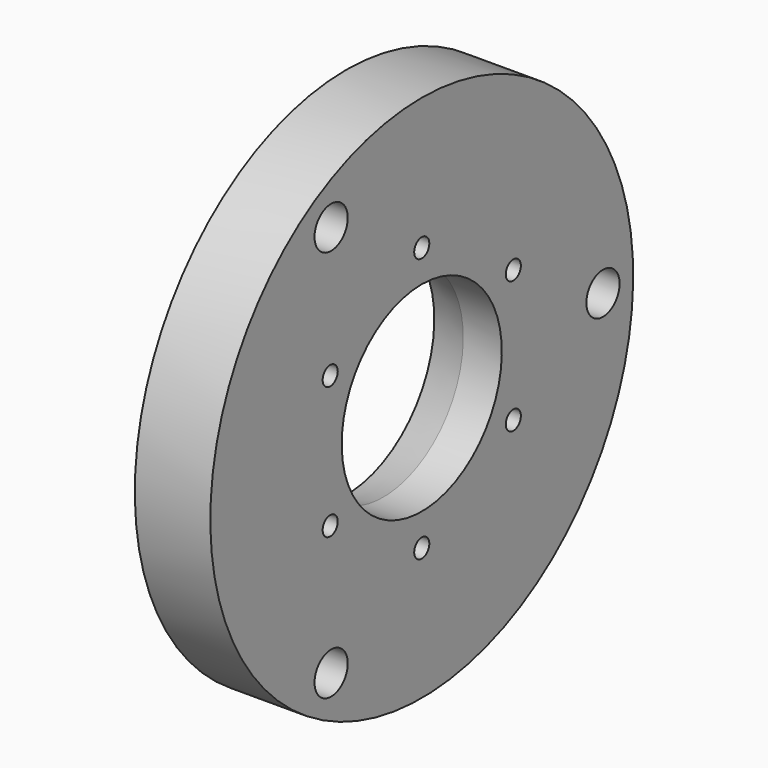
from build123d import *

# Parameters (mm, degrees)
F2_R            = 5.5
F3_DEPTH        = 20.001
F3_COPIES_COUNT = 3
F4_R            = 2.5
F5_DEPTH        = 15
F5_COPIES_COUNT = 6


# Not quite as in the source:
# - a pattern or mirror of a feature is missing from the dataset's text; its kind, count and spacing are read off the source's solid


with BuildPart() as f1:
    # F0 (on Front) → F1 (revolve)
    with BuildSketch(Plane.XZ):
        Polygon((0, 70), (0, 29.148), (9.798351825, 26.5), (20, 26.5), (20, 70), align=None)
    revolve(axis=Axis((21.5308236951, 0, 0), (1, 0, 0)))

    # F2 (on face) → F3 (cut, through all)
    with BuildSketch(Plane(origin=(0, 0, 0), x_dir=(0, -1, 0), z_dir=(-1, 0, 0))):
        with Locations((30, 51.9615242271)):
            Circle(F2_R)
    f3 = extrude(amount=-F3_DEPTH, mode=Mode.SUBTRACT)

    # F3_copies: F3 ×3 about axis
    f3_copies_axis = Axis((0, 0, 0), (1, 0, 0))
    for i in range(1, F3_COPIES_COUNT):
        add(f3.rotate(f3_copies_axis, i * 360 / F3_COPIES_COUNT), mode=Mode.SUBTRACT)

    # F4 (on face) → F5 (cut)
    with BuildSketch(Plane.YZ.offset(20)):
        with Locations((-30.3108891325, 17.5)):
            Circle(F4_R)
    f5 = extrude(amount=-F5_DEPTH, mode=Mode.SUBTRACT)

    # F5_copies: F5 ×6 about axis
    f5_copies_axis = Axis((0, 0, 0), (1, 0, 0))
    for i in range(1, F5_COPIES_COUNT):
        add(f5.rotate(f5_copies_axis, i * 360 / F5_COPIES_COUNT), mode=Mode.SUBTRACT)


solid = f1.part
